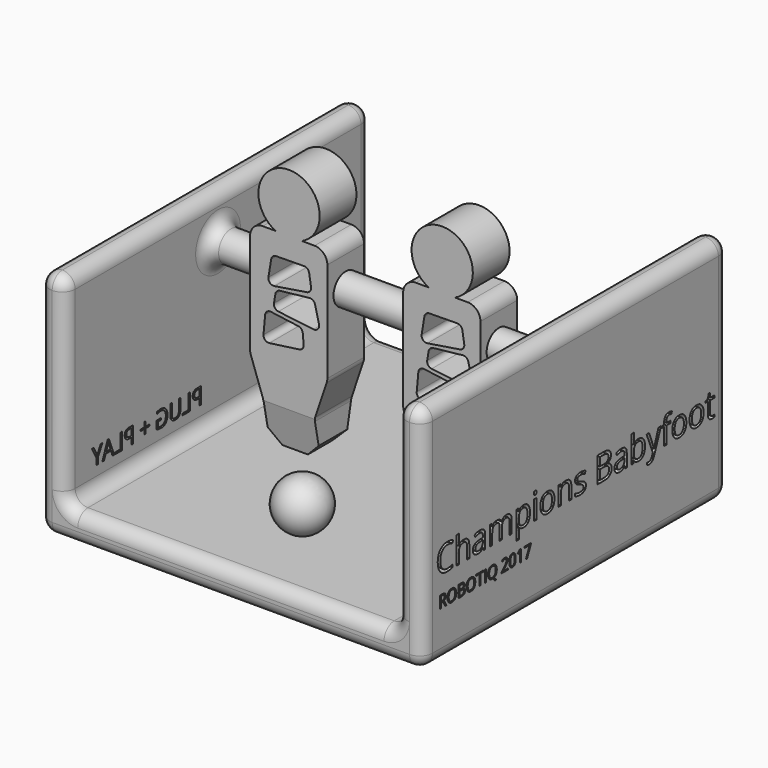
from build123d import *

# Parameters (mm, degrees)
F1_DEPTH        = 9
F2_R            = 5
F2_2_R          = 5
F3_SIZE         = 5
F3_2_SIZE       = 5
F4_C1_SIZE2     = 3
F4_C1_SIZE      = 15
F4_C2_SIZE2     = 3
F4_C2_SIZE      = 15
F4_2_C1_SIZE2   = 3
F4_2_C1_SIZE    = 15
F4_2_C2_SIZE2   = 3
F4_2_C2_SIZE    = 15
F5_R            = 6
F6_DEPTH        = 75
F10_DEPTH       = 75
F11_R           = 4.99999
F12_TEXT_SIZE   = 13.9975545204
F12_TEXT_SIZE_2 = 6.5321920879
F13_DEPTH       = 25
F15_DEPTH       = 25
F16_R           = 2
F18_DEPTH       = 25
F19_R           = 2
F20_TEXT_SIZE   = 9.0726637182
F21_DEPTH       = 25
F24_W           = 8.1040523946
F24_H           = 0.3642197698
F24_W_2         = 5.1115825772
F24_H_2         = 0.4259650595
F25_DEPTH       = 1
F27_W           = 6.1979177408
F27_H           = 0.7151449099
F27_W_2         = 5.3039863706
F27_H_2         = 0.5959542468
F27_W_3         = 4.41005826
F28_DEPTH       = 1


# Not quite as in the source:
# - a fillet or chamfer is up to 0.001 mm smaller than in the source, because OpenCascade refuses the exact size
# - Text() gives the source's letters only with a copy of the font that has no kerning and outlines rounded to 1/6400 em; it was checked with that copy


with BuildPart() as f1:
    # F0 (on Front) → F1 (new body, symmetric)
    with BuildSketch(Plane.XZ):
        with BuildLine():
            Line((-45.2903602755, 30), (-40, 15))
            Line((-40, 15), (-40, 0))
            Line((-40, 0), (-30, 0))
            Line((-30, 0), (-20, 0))
            Line((-20, 0), (-20, 15))
            Line((-20, 15), (-15, 29.8621786635))
            Line((-15, 29.8621786635), (-15, 74.8621786635))
            Line((-15, 74.8621786635), (-25, 74.8621786635))
            ThreePointArc((-25, 74.8621786635), (-29.8392954494, 97.7698146486), (-35.2903602755, 75))
            Line((-35.2903602755, 75), (-45.2903602755, 75))
            Line((-45.2903602755, 75), (-45.2903602755, 30))
        make_face()
    extrude(amount=F1_DEPTH, both=True)

    # F2
    f2_edges = [f1.edges().sort_by_distance(p)[0] for p in [
        (-45.29036, 0, 75),
        (-45.29036, 0, 30),
        (-40, 0, 15),
        (-15, 0, 74.862179),
        (-15, 0, 29.862179),
        (-20, 0, 15),
    ]]
    fillet(f2_edges, radius=F2_R)

    # F3
    f3_edges = [f1.edges().sort_by_distance(p)[0] for p in [
        (-40, 0, 0),
        (-20, 0, 0),
    ]]
    chamfer(f3_edges, length=F3_SIZE)

    # F4: chamfer of 15 x 3 on 3 edges, made by hand

    # F4_c1
    f4_c1_edges = [f1.edges().sort_by_distance(p)[0] for p in [
        (-30, 9, 0),
    ]]
    f4_c1_side = f1.faces().sort_by_distance((-30, 9, 0.06))[0]
    chamfer(f4_c1_edges, length=F4_C1_SIZE, length2=F4_C1_SIZE2, reference=f4_c1_side)

    # F4_c2
    f4_c2_edges = [f1.edges().sort_by_distance(p)[0] for p in [
        (-30, -9, 0),
    ]]
    f4_c2_side = f1.faces().sort_by_distance((-30, -9, 0.06))[0]
    chamfer(f4_c2_edges, length=F4_C2_SIZE, length2=F4_C2_SIZE2, reference=f4_c2_side)



with BuildPart() as f1b:
    # F0 (on Front) → F1, piece 2 (new body, symmetric)
    with BuildSketch(Plane.XZ):
        with BuildLine():
            Line((14.7096397245, 30), (20, 15))
            Line((20, 15), (20, 0))
            Line((20, 0), (30, 0))
            Line((30, 0), (40, 0))
            Line((40, 0), (40, 15))
            Line((40, 15), (45, 29.8621786635))
            Line((45, 29.8621786635), (45, 74.8621786635))
            Line((45, 74.8621786635), (35, 74.8621786635))
            ThreePointArc((35, 74.8621786635), (30.1607045506, 97.7698146486), (24.7096397245, 75))
            Line((24.7096397245, 75), (14.7096397245, 75))
            Line((14.7096397245, 75), (14.7096397245, 30))
        make_face()
    extrude(amount=F1_DEPTH, both=True)

    # F2#2
    f2_2_edges = [f1b.edges().sort_by_distance(p)[0] for p in [
        (20, 0, 15),
        (14.70964, 0, 30),
        (14.70964, 0, 75),
        (40, 0, 15),
        (45, 0, 29.862179),
        (45, 0, 74.862179),
    ]]
    fillet(f2_2_edges, radius=F2_2_R)

    # F3#2
    f3_2_edges = [f1b.edges().sort_by_distance(p)[0] for p in [
        (40, 0, 0),
        (20, 0, 0),
    ]]
    chamfer(f3_2_edges, length=F3_2_SIZE)

    # F4#2: chamfer of 15 x 3 on 3 edges, made by hand

    # F4_2_c1
    f4_2_c1_edges = [f1b.edges().sort_by_distance(p)[0] for p in [
        (30, 9, 0),
    ]]
    f4_2_c1_side = f1b.faces().sort_by_distance((30, 9, 0.06))[0]
    chamfer(f4_2_c1_edges, length=F4_2_C1_SIZE, length2=F4_2_C1_SIZE2, reference=f4_2_c1_side)

    # F4_2_c2
    f4_2_c2_edges = [f1b.edges().sort_by_distance(p)[0] for p in [
        (30, -9, 0),
    ]]
    f4_2_c2_side = f1b.faces().sort_by_distance((30, -9, 0.06))[0]
    chamfer(f4_2_c2_edges, length=F4_2_C2_SIZE, length2=F4_2_C2_SIZE2, reference=f4_2_c2_side)


with BuildPart() as f1_1:
    add(f1.part)

    add(f1b.part)  # F6 merges F1b
    # F5 (on Right) → F6 (join, symmetric)
    with BuildSketch(Plane.YZ):
        with Locations((0, 58)):
            Circle(F5_R)
    extrude(amount=F6_DEPTH, both=True)

    # F9 (on Front) → F10 (join, symmetric)
    with BuildSketch(Plane.XZ):
        Polygon((-75, 75), (-75, -15), (75, -15), (75, 75), (65, 75), (65, 0), (65, -3.7155121099), (-65, -3.7155121099), (-65, 1.1136030793), (-65, 75), align=None)
    extrude(amount=F10_DEPTH, both=True)

    # F11 (radius 5 in the source; OpenCascade refuses exactly that, so slightly less here)
    f11_edges = [f1_1.edges().sort_by_distance(p)[0] for p in [
        (-75, 0, 75),
        (-70, -75, 75),
        (-70, 75, 75),
        (-65, 0, 75),
        (-65, 75, 35.642244),
        (-75, 75, 30),
        (-75, -75, 30),
        (-65, -75, 35.642244),
        (0, -75, -3.715512),
        (0, -75, -15),
        (-75, 0, -15),
        (0, 75, -15),
        (75, 0, -15),
        (75, -75, 30),
        (65, -75, 35.642244),
        (75, 75, 30),
        (65, 75, 35.642244),
        (0, 75, -3.715512),
        (70, 75, 75),
        (75, 0, 75),
        (65, 0, 75),
        (-65, 0, -3.715512),
        (65, 0, -3.715512),
        (65, -6, 58),
        (70, -75, 75),
        (-65, -6, 58),
    ]]
    fillet(f11_edges, radius=F11_R)

    # F12 (on face) → F13 (cut)
    with BuildSketch(Plane.YZ.offset(75)):
        with Locations((-68.2910652831, 15.3580578044)):
            Text('Champions Babyfoot', F12_TEXT_SIZE, font='Open Sans', text_align=(TextAlign.LEFT, TextAlign.BOTTOM))
        with Locations((-67.0762807131, 3.7702347618)):
            Text('ROBOTIQ 2017', F12_TEXT_SIZE_2, font='Open Sans', text_align=(TextAlign.LEFT, TextAlign.BOTTOM))
    extrude(amount=-F13_DEPTH, mode=Mode.SUBTRACT)

    # F14 (on face) → F15 (cut)
    with BuildSketch(Plane(origin=(-75, 0, 0), x_dir=(0, -1, 0), z_dir=(-1, 0, 0))):
        Polygon((-28.8373369213, 51.5991695779), (-43.1635305285, 51.4286197722), (-44.9552163482, 40.4545404017), (-27.5050215423, 43.2337336242), align=None)
        Polygon((-26.6790315509, 41.4571948349), (-41.5447428823, 39.8279353976), (-42.6645465195, 32.8851491213), (-23.9957235754, 30.6117516011), align=None)
        Polygon((-31.2099158764, 29.9179852009), (-45.6178708508, 31.8721102247), (-46.6690212488, 20.2425401658), (-30.5283833295, 22.4806908518), align=None)
    extrude(amount=-F15_DEPTH, mode=Mode.SUBTRACT)

    # F16
    f16_edges = [f1_1.edges().sort_by_distance(p)[0] for p in [
        (-70, 23.995724, 30.611752),
        (-70, 26.679032, 41.457195),
        (-70, 42.664547, 32.885149),
        (-70, 41.544743, 39.827935),
        (-70, 45.617871, 31.87211),
        (-70, 31.209916, 29.917985),
        (-70, 30.528383, 22.480691),
        (-70, 46.669021, 20.24254),
        (-70, 27.505022, 43.233734),
        (-70, 28.837337, 51.59917),
        (-70, 44.955216, 40.45454),
        (-70, 43.163531, 51.42862),
    ]]
    fillet(f16_edges, radius=F16_R)

    # F17 (on face) → F18 (cut)
    with BuildSketch(Plane.XZ.offset(9)):
        Polygon((-22.4040697749, 66.5106665897), (-36.7302633822, 66.340116784), (-38.5219492018, 55.3660374135), (-21.071754396, 58.145230636), align=None)
        Polygon((-20.2457644045, 56.3686918467), (-35.1114757359, 54.7394324094), (-36.2312793732, 47.7966461331), (-17.562456429, 45.5232486129), align=None)
        Polygon((-24.77664873, 44.8294822127), (-39.1846037044, 46.7836072364), (-40.2357541025, 35.1540371776), (-24.0951161832, 37.3921878636), align=None)
        Polygon((37.6235572355, 66.2908637342), (23.2973636283, 66.1203139286), (21.5056778087, 55.1462345581), (38.9558726145, 57.9254277806), align=None)
        Polygon((39.7818626059, 56.1488889913), (24.9161512746, 54.519629554), (23.7963476373, 47.5768432776), (42.4651705815, 45.3034457575), align=None)
        Polygon((35.2509782804, 44.6096793572), (20.843023306, 46.563804381), (19.791872908, 34.9342343221), (35.9325108273, 37.1723850082), align=None)
    extrude(amount=-F18_DEPTH, mode=Mode.SUBTRACT)

    # F19
    f19_edges = [f1_1.edges().sort_by_distance(p)[0] for p in [
        (-36.730263, 0, 66.340117),
        (-35.111476, 0, 54.739432),
        (-39.184604, 0, 46.783607),
        (-22.40407, 0, 66.510667),
        (-20.245764, 0, 56.368692),
        (-24.776649, 0, 44.829482),
        (35.250978, 0, 44.609679),
        (39.781863, 0, 56.148889),
        (37.623557, 0, 66.290864),
        (20.843023, 0, 46.563804),
        (24.916151, 0, 54.51963),
        (23.297364, 0, 66.120314),
        (19.791873, 0, 34.934234),
        (23.796348, 0, 47.576843),
        (21.505678, 0, 55.146235),
        (-36.231279, 0, 47.796646),
        (-40.235754, 0, 35.154037),
        (-38.521949, 0, 55.366037),
        (-21.071754, 0, 58.145231),
        (-17.562456, 0, 45.523249),
        (-24.095116, 0, 37.392188),
        (35.932511, 0, 37.172385),
        (42.465171, 0, 45.303446),
        (38.955873, 0, 57.925428),
    ]]
    fillet(f19_edges, radius=F19_R)

    # F20 (on face) → F21 (cut)
    with BuildSketch(Plane(origin=(-75, 0, 0), x_dir=(0, -1, 0), z_dir=(-1, 0, 0))):
        with Locations((7.4643054977, 5.1140002906)):
            Text('PLUG + PLAY', F20_TEXT_SIZE, font='Open Sans', text_align=(TextAlign.LEFT, TextAlign.BOTTOM))
    extrude(amount=-F21_DEPTH, mode=Mode.SUBTRACT)

    # F8 (on offset) → F22 (revolve)
    with BuildSketch(Plane.XZ.offset(40)):
        with BuildLine():
            ThreePointArc((10, 4.9258163199), (0, 14.9258163199), (-10, 4.9258163199))
            Line((-10, 4.9258163199), (10, 4.9258163199))
        make_face()
    revolve(axis=Axis((0, -40, 4.9258163199), (1, 0, 0)))

    # F24 (on offset) → F25 (join, symmetric)
    with BuildSketch(Plane.YZ.offset(70)):
        with Locations((-46.9418745488, 17.8638221696)):
            Rectangle(F24_W, F24_H)
        with Locations((-25.7406160235, 19.4216603413)):
            Rectangle(F24_W, F24_H)
        with Locations((-13.8129135594, 18.6685714871)):
            Rectangle(F24_W, F24_H)
        with Locations((22.4799746647, 17.5790116191)):
            Rectangle(F24_W, F24_H)
        with Locations((50.9644690901, 18.8183439896)):
            Rectangle(F24_W, F24_H)
        with Locations((59.568522498, 18.8183439896)):
            Rectangle(F24_W, F24_H)
        with Locations((30.5436532944, 19.0690094605)):
            Rectangle(F24_W, F24_H)
        with Locations((13.9452274889, 18.0888613686)):
            Rectangle(F24_W, F24_H)
        with Locations((14.2567455769, 22.6775882766)):
            Rectangle(F24_W, F24_H)
        with Locations((-60.4298077524, 5.6309953798)):
            Rectangle(F24_W_2, F24_H_2)
        with Locations((-55.5728748441, 4.9168774858)):
            Rectangle(F24_W_2, F24_H_2)
        with Locations((-55.8973290026, 7.6519262511)):
            Rectangle(F24_W_2, F24_H_2)
        with Locations((-51.3557456434, 6.3719262835)):
            Rectangle(F24_W_2, F24_H_2)
        with Locations((-65.3051026165, 7.3111827951)):
            Rectangle(F24_W_2, F24_H_2)
        with Locations((-40.8013090491, 6.0872030444)):
            Rectangle(F24_W_2, F24_H_2)
        with Locations((-30.5929332972, 5.9198017698)):
            Rectangle(F24_W_2, F24_H_2)
    extrude(amount=F25_DEPTH, both=True)

    # F27 (on offset) → F28 (join, symmetric)
    with BuildSketch(Plane(origin=(-70, 0, 0), x_dir=(0, -1, 0), z_dir=(-1, 0, 0))):
        with Locations((10.016848566, 9.5870862715)):
            Rectangle(F27_W, F27_H)
        with Locations((43.6584353447, 9.5274909399)):
            Rectangle(F27_W_2, F27_H_2)
        with Locations((53.7598505616, 9.5274909399)):
            Rectangle(F27_W_3, F27_H_2)
    extrude(amount=F28_DEPTH, both=True)


solid = f1_1.part
